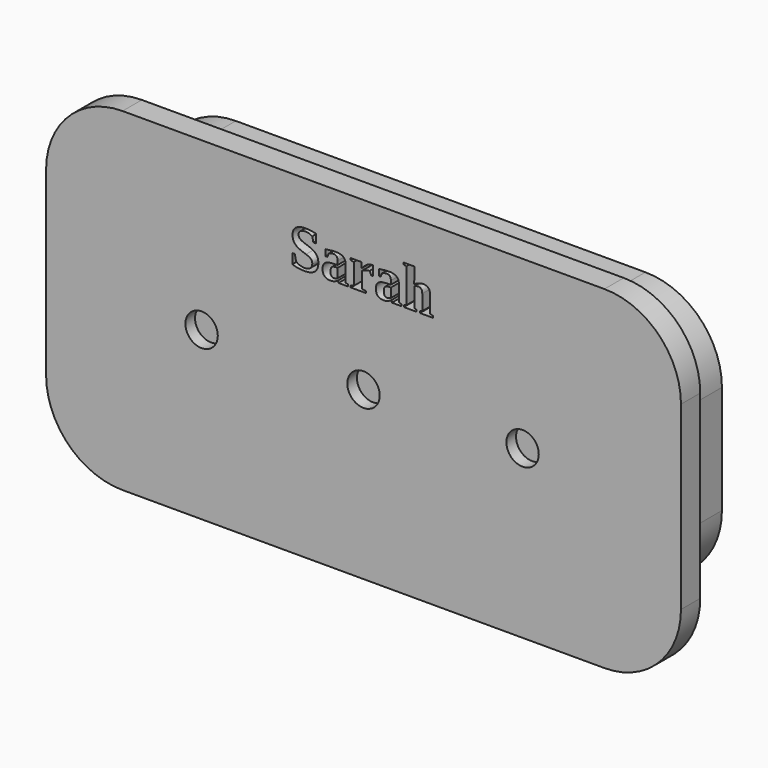
from build123d import *

# Parameters (mm, degrees)
F1_DEPTH     = 2
F2_R         = 1.3437672095
F3_DEPTH     = 1
F5_DEPTH     = 6
F6_TEXT_SIZE = 4.6867463324
F7_DEPTH     = 2


# Not quite as in the source:
# - Text() gives the source's letters only with a copy of the font that has no kerning and outlines rounded to 1/6400 em; it was checked with that copy


with BuildPart() as f1:
    # F0 (on Front) → F1 (new body)
    with BuildSketch(Plane.XZ):
        with BuildLine():
            Line((-20, -13.85), (20, -13.85))
            ThreePointArc((20, -13.85), (24.4901280605, -11.9901280605), (26.35, -7.5))
            Line((26.35, -7.5), (26.35, 7.5))
            ThreePointArc((26.35, 7.5), (24.4901280605, 11.9901280605), (20, 13.85))
            Line((20, 13.85), (-20, 13.85))
            ThreePointArc((-20, 13.85), (-24.4901280605, 11.9901280605), (-26.35, 7.5))
            Line((-26.35, 7.5), (-26.35, -7.5))
            ThreePointArc((-26.35, -7.5), (-24.4901280605, -11.9901280605), (-20, -13.85))
        make_face()
    extrude(amount=F1_DEPTH)

    # F2 (on face) → F3 (cut)
    with BuildSketch(Plane.XZ.offset(2)):
        with Locations((-13.4405605495, 0)):
            Circle(F2_R)
        Circle(F2_R)
        with Locations((13.2037326694, 0)):
            Circle(F2_R)
    extrude(amount=-F3_DEPTH, mode=Mode.SUBTRACT)

    # F4 (on face) → F5 (join)
    with BuildSketch(Plane(origin=(0, 0, 0), x_dir=(-1, 0, 0), z_dir=(0, 1, 0))):
        with BuildLine():
            Line((-17, -10.85), (17, -10.85))
            ThreePointArc((17, -10.85), (21.4901280605, -8.9901280605), (23.35, -4.5))
            Line((23.35, -4.5), (23.35, 4.5))
            ThreePointArc((23.35, 4.5), (21.4901280605, 8.9901280605), (17, 10.85))
            Line((17, 10.85), (-17, 10.85))
            ThreePointArc((-17, 10.85), (-21.4901280605, 8.9901280605), (-23.35, 4.5))
            Line((-23.35, 4.5), (-23.35, -4.5))
            ThreePointArc((-23.35, -4.5), (-21.4901280605, -8.9901280605), (-17, -10.85))
        make_face()
    extrude(amount=F5_DEPTH)

    # F6 (on face) → F7 (cut)
    with BuildSketch(Plane.XZ.offset(2)):
        with Locations((-6.1574318515, 7.1148891002)):
            Text('Sarah', F6_TEXT_SIZE, font='Tinos', font_style=FontStyle.BOLD, text_align=(TextAlign.LEFT, TextAlign.BOTTOM))
    extrude(amount=-F7_DEPTH, mode=Mode.SUBTRACT)


solid = f1.part
